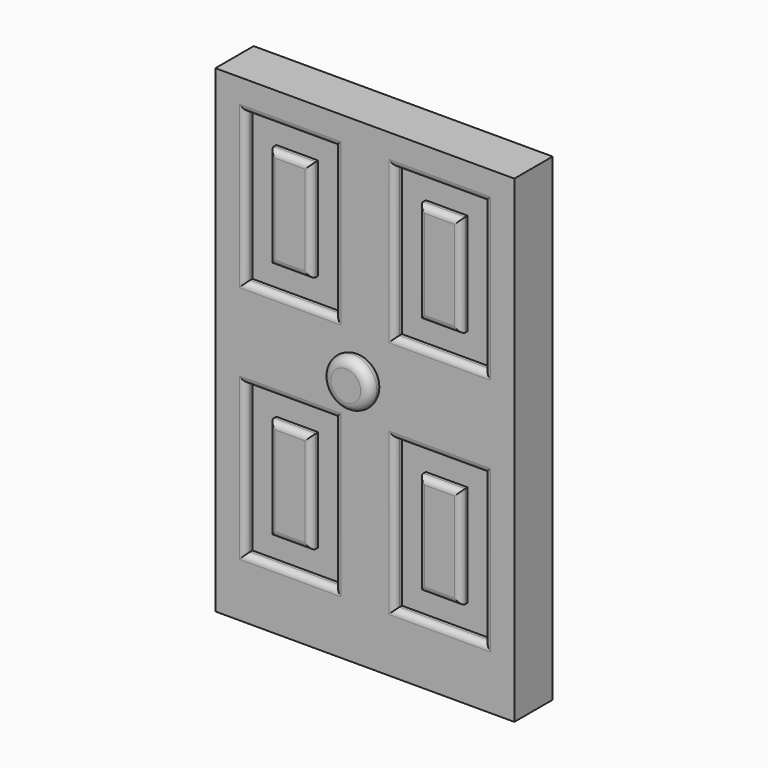
from build123d import *

# Parameters (mm, degrees)
F0_W     = 50
F0_H     = 80
F1_DEPTH = 8
F2_W     = 15
F2_H     = 25
F2_W_2   = 7
F2_H_2   = 17
F3_DEPTH = 1.5
F4_R     = 1
F5_R     = 2
F6_DEPTH = 1
F7_R     = 4
F7_R_2   = 2
F8_DEPTH = 3
F9_R     = 1.49999


# Not quite as in the source:
# - a fillet or chamfer is up to 0.001 mm smaller than in the source, because OpenCascade refuses the exact size


with BuildPart() as f1:
    # F0 (on Front) → F1 (new body)
    with BuildSketch(Plane.XZ):
        with Locations((25, 40)):
            Rectangle(F0_W, F0_H)
    extrude(amount=F1_DEPTH)

    # F2 (on face) → F3 (cut)
    with BuildSketch(Plane.XZ.offset(8)):
        with Locations((12.5, 62.5)):
            Rectangle(F2_W, F2_H)
        with Locations((12.5, 62.5)):
            Rectangle(F2_W_2, F2_H_2, mode=Mode.SUBTRACT)
        with Locations((37.5, 62.5)):
            Rectangle(F2_W, F2_H)
        with Locations((37.5, 62.5)):
            Rectangle(F2_W_2, F2_H_2, mode=Mode.SUBTRACT)
        with Locations((12.5, 22.5)):
            Rectangle(F2_W, F2_H)
        with Locations((12.5, 22.5)):
            Rectangle(F2_W_2, F2_H_2, mode=Mode.SUBTRACT)
        with Locations((37.5, 22.5)):
            Rectangle(F2_W, F2_H)
        with Locations((37.5, 22.5)):
            Rectangle(F2_W_2, F2_H_2, mode=Mode.SUBTRACT)
    extrude(amount=-F3_DEPTH, mode=Mode.SUBTRACT)

    # F4
    f4_edges = [f1.edges().sort_by_distance(p)[0] for p in [
        (16, -8, 62.5),
        (12.5, -8, 71),
        (9, -8, 62.5),
        (12.5, -8, 54),
        (5, -8, 62.5),
        (12.5, -8, 75),
        (20, -8, 62.5),
        (12.5, -8, 50),
        (37.5, -8, 75),
        (45, -8, 62.5),
        (37.5, -8, 71),
        (30, -8, 62.5),
        (34, -8, 62.5),
        (41, -8, 62.5),
        (37.5, -8, 54),
        (37.5, -8, 50),
        (37.5, -8, 35),
        (37.5, -8, 31),
        (34, -8, 22.5),
        (37.5, -8, 14),
        (41, -8, 22.5),
        (45, -8, 22.5),
        (37.5, -8, 10),
        (30, -8, 22.5),
        (20, -8, 22.5),
        (16, -8, 22.5),
        (9, -8, 22.5),
        (5, -8, 22.5),
        (12.5, -8, 35),
        (12.5, -8, 31),
        (12.5, -8, 14),
        (12.5, -8, 10),
    ]]
    fillet(f4_edges, radius=F4_R)

    # F5 (on face) → F6 (join)
    with BuildSketch(Plane.XZ.offset(8)):
        with Locations((25, 43)):
            Circle(F5_R)
    extrude(amount=F6_DEPTH)

    # F7 (on face) → F8 (join)
    with BuildSketch(Plane.XZ.offset(9)):
        with Locations((25, 43)):
            Circle(F7_R)
        with Locations((25, 43)):
            Circle(F7_R_2, mode=Mode.SUBTRACT)
        with Locations((25, 43)):
            Circle(F7_R_2)
    extrude(amount=F8_DEPTH)

    # F9 (radius 1.5 in the source; OpenCascade refuses exactly that, so slightly less here)
    f9_edges = [f1.edges().sort_by_distance(p)[0] for p in [
        (21, -12, 43),
        (21, -9, 43),
    ]]
    fillet(f9_edges, radius=F9_R)


solid = f1.part
